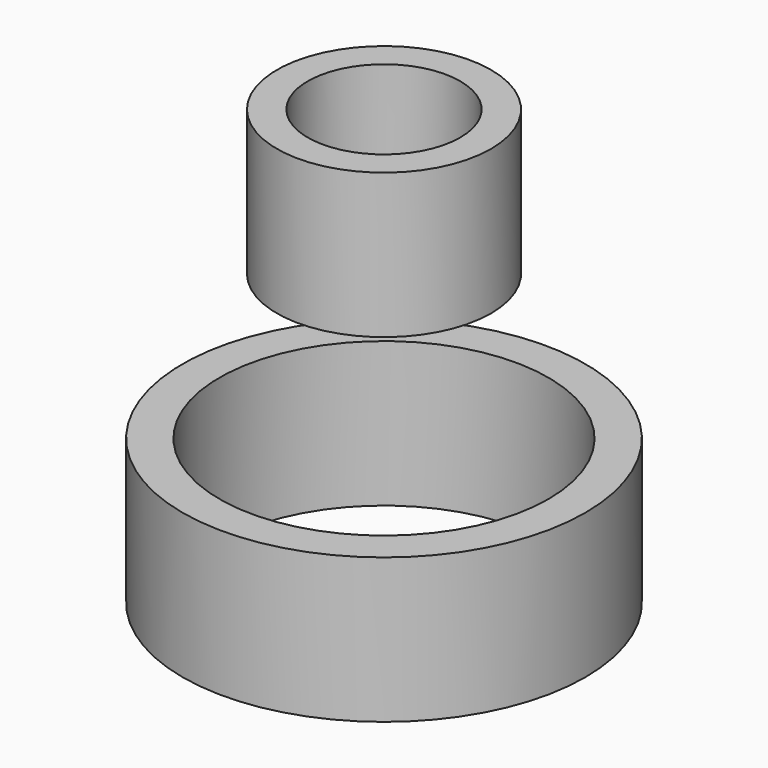
from build123d import *

# Parameters (mm, degrees)
F0_R     = 35.3264234519
F0_R_2   = 28.8496672687
F1_DEPTH = 25.4
F3_R     = 18.7767042544
F3_R_2   = 13.3768660961
F4_DEPTH = 25.4


# Not quite as in the source:
# - the program builds the solid bodies; features that only make, move or delete a surface that nothing else refers to are left out


with BuildPart() as f1:
    # F0 (on Top) → F1 (new body)
    with BuildSketch(Plane.XY):
        Circle(F0_R)
        Circle(F0_R_2, mode=Mode.SUBTRACT)
    extrude(amount=F1_DEPTH)


with BuildPart() as f4:
    # F3 (on offset) → F4 (new body)
    with BuildSketch(Plane.XY.offset(50.8)):
        Circle(F3_R)
        Circle(F3_R_2, mode=Mode.SUBTRACT)
    extrude(amount=F4_DEPTH)


solid = Compound([f1.part, f4.part])
